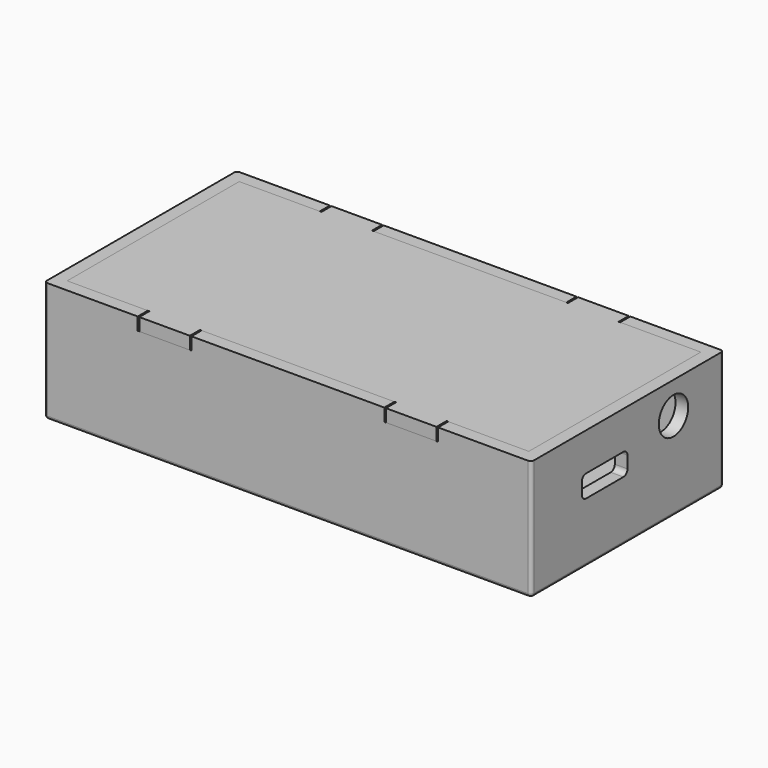
from build123d import *

# Parameters (mm, degrees)
F0_W         = 73
F0_H         = 34
F1_DEPTH     = 17
F2_T         = 2
F3_W         = 9
F3_H         = 3.5
F4_DEPTH     = 25.4
F5_R         = 2.905
F6_DEPTH     = 25.4
F7_R         = 0.8
F8_T1_DEPTH  = 37
F8_T3_DEPTH  = 19.75
F8_T5_DEPTH  = 76
F8_S9_W      = 0.51
F8_S9_H      = 0.51
F8_T10_DEPTH = 0.51
F8_S15_W     = 0.51
F8_S15_H     = 0.51
F8_T16_DEPTH = 0.51
F8_S21_W     = 0.51
F8_S21_H     = 0.51
F8_T22_DEPTH = 0.51
F8_S27_W     = 0.51
F8_S27_H     = 0.51
F8_T28_DEPTH = 0.51
F9_W         = 8.5
F9_H         = 2
F10_DEPTH    = 2
F12_DEPTH    = 2
F13_W        = 8
F13_H        = 1.5
F14_DEPTH    = 9.5
F16_DEPTH    = 1.5


# Not quite as in the source:
# - a fillet or chamfer that OpenCascade refuses, or shapes differently, is made with other operations: its cross-section is extruded or revolved along the edge and cut away or added


with BuildPart() as f1:
    # F0 (on Top) → F1 (new body)
    with BuildSketch(Plane.XY):
        with Locations((36.5, 17)):
            Rectangle(F0_W, F0_H)
    extrude(amount=F1_DEPTH)

    # F2
    f2_openings = [f1.faces().sort_by_distance(p)[0] for p in [
        (36.5, 17, 17),
    ]]
    offset(amount=F2_T, openings=f2_openings, kind=Kind.INTERSECTION)

    # F3 (on face) → F4 (cut)
    with BuildSketch(Plane.YZ.offset(75)):
        with Locations((12.5, 9.25)):
            Rectangle(F3_W, F3_H)
    extrude(amount=-F4_DEPTH, mode=Mode.SUBTRACT)

    # F5 (on face) → F6 (cut)
    with BuildSketch(Plane.YZ.offset(75)):
        with Locations((26.095, 12)):
            Circle(F5_R)
    extrude(amount=-F6_DEPTH, mode=Mode.SUBTRACT)

    # F7
    f7_edges = [f1.edges().sort_by_distance(p)[0] for p in [
        (74, 8, 7.5),
        (74, 17, 11),
        (74, 17, 7.5),
        (74, 8, 11),
    ]]
    fillet(f7_edges, radius=F7_R)

    # F8: fillet of radius 0.5 on 9 edges, made by hand

    # F8_s2 → F8_t1 (cut)
    with BuildSketch(Plane.XZ.offset(-35.5)):
        with BuildLine():
            ThreePointArc((75, -1.5), (74.8535533906, -1.8535533906), (74.5, -2))
            Line((74.5, -2), (75, -2))
            Line((75, -2), (75, -1.5))
        make_face()
        with BuildLine():
            ThreePointArc((-2, -1.5), (-1.8535533906, -1.8535533906), (-1.5, -2))
            Line((-1.5, -2), (-2, -2))
            Line((-2, -2), (-2, -1.5))
        make_face()
    extrude(amount=F8_T1_DEPTH, mode=Mode.SUBTRACT)

    # F8_s4 → F8_t3 (cut)
    with BuildSketch(Plane.XY.offset(-1.5)):
        with BuildLine():
            ThreePointArc((75, -1.5), (74.8535533906, -1.8535533906), (74.5, -2))
            Line((74.5, -2), (75, -2))
            Line((75, -2), (75, -1.5))
        make_face()
        with BuildLine():
            ThreePointArc((75, 35.5), (74.8535533906, 35.8535533906), (74.5, 36))
            Line((74.5, 36), (75, 36))
            Line((75, 36), (75, 35.5))
        make_face()
        with BuildLine():
            ThreePointArc((-1.5, 36), (-1.8535533906, 35.8535533906), (-2, 35.5))
            Line((-2, 35.5), (-2, 36))
            Line((-2, 36), (-1.5, 36))
        make_face()
        with BuildLine():
            ThreePointArc((-2, -1.5), (-1.8535533906, -1.8535533906), (-1.5, -2))
            Line((-1.5, -2), (-2, -2))
            Line((-2, -2), (-2, -1.5))
        make_face()
    extrude(amount=F8_T3_DEPTH, mode=Mode.SUBTRACT)

    # F8_s6 → F8_t5 (cut)
    with BuildSketch(Plane.YZ.offset(-1.5)):
        with BuildLine():
            ThreePointArc((36, -1.5), (35.8535533906, -1.8535533906), (35.5, -2))
            Line((35.5, -2), (36, -2))
            Line((36, -2), (36, -1.5))
        make_face()
        with BuildLine():
            ThreePointArc((-2, -1.5), (-1.8535533906, -1.8535533906), (-1.5, -2))
            Line((-1.5, -2), (-2, -2))
            Line((-2, -2), (-2, -1.5))
        make_face()
    extrude(amount=F8_T5_DEPTH, mode=Mode.SUBTRACT)


with BuildPart() as f8_tool8:
    # F8_s9 → F8_t10 (new body)
    with BuildSketch(Plane.XZ.offset(1.5)):
        with Locations((74.755, -1.755)):
            Rectangle(F8_S9_W, F8_S9_H)
    extrude(amount=F8_T10_DEPTH)

    # F8_s11 → F8_t12 (revolve, cut)
    with BuildSketch(Plane(origin=(74.5, -1.5, -1.5), x_dir=(-0.7071067812, 0, 0.7071067812), z_dir=(0.7071067812, 0, 0.7071067812))):
        with BuildLine():
            ThreePointArc((0, -0.5), (0.5, 0), (0, 0.5))
            Line((0, 0.5), (0, -0.5))
        make_face()
    revolve(axis=Axis((74.5, -1.5, -1.5), (0, -1, 0)), mode=Mode.SUBTRACT)


with BuildPart() as f1_1:
    add(f1.part)

    # F8_t7: cut F8_tool8
    add(f8_tool8.part, mode=Mode.SUBTRACT)


with BuildPart() as f8_tool14:
    # F8_s15 → F8_t16 (new body)
    with BuildSketch(Plane.XZ.offset(-35.5)):
        with Locations((74.755, -1.755)):
            Rectangle(F8_S15_W, F8_S15_H)
    extrude(amount=-F8_T16_DEPTH)

    # F8_s17 → F8_t18 (revolve, cut)
    with BuildSketch(Plane(origin=(74.5, 35.5, -1.5), x_dir=(-0.7071067812, 0, 0.7071067812), z_dir=(-0.7071067812, 0, -0.7071067812))):
        with BuildLine():
            ThreePointArc((0, -0.5), (0.5, 0), (0, 0.5))
            Line((0, 0.5), (0, -0.5))
        make_face()
    revolve(axis=Axis((74.5, 35.5, -1.5), (0, 1, 0)), mode=Mode.SUBTRACT)


with BuildPart() as f1_2:
    add(f1_1.part)

    # F8_t13: cut F8_tool14
    add(f8_tool14.part, mode=Mode.SUBTRACT)


with BuildPart() as f8_tool20:
    # F8_s21 → F8_t22 (new body)
    with BuildSketch(Plane.XZ.offset(-35.5)):
        with Locations((-1.755, -1.755)):
            Rectangle(F8_S21_W, F8_S21_H)
    extrude(amount=-F8_T22_DEPTH)

    # F8_s23 → F8_t24 (revolve, cut)
    with BuildSketch(Plane(origin=(-1.5, 35.5, -1.5), x_dir=(0.7071067812, 0, 0.7071067812), z_dir=(-0.7071067812, 0, 0.7071067812))):
        with BuildLine():
            ThreePointArc((0, -0.5), (0.5, 0), (0, 0.5))
            Line((0, 0.5), (0, -0.5))
        make_face()
    revolve(axis=Axis((-1.5, 35.5, -1.5), (0, 1, 0)), mode=Mode.SUBTRACT)


with BuildPart() as f1_3:
    add(f1_2.part)

    # F8_t19: cut F8_tool20
    add(f8_tool20.part, mode=Mode.SUBTRACT)


with BuildPart() as f8_tool26:
    # F8_s27 → F8_t28 (new body)
    with BuildSketch(Plane.YZ.offset(-1.5)):
        with Locations((-1.755, -1.755)):
            Rectangle(F8_S27_W, F8_S27_H)
    extrude(amount=-F8_T28_DEPTH)

    # F8_s29 → F8_t30 (revolve, cut)
    with BuildSketch(Plane(origin=(-1.5, -1.5, -1.5), x_dir=(0, 0.7071067812, 0.7071067812), z_dir=(0, -0.7071067812, 0.7071067812))):
        with BuildLine():
            ThreePointArc((0, -0.5), (0.5, 0), (0, 0.5))
            Line((0, 0.5), (0, -0.5))
        make_face()
    revolve(axis=Axis((-1.5, -1.5, -1.5), (-1, 0, 0)), mode=Mode.SUBTRACT)


with BuildPart() as f1_4:
    add(f1_3.part)

    # F8_t25: cut F8_tool26
    add(f8_tool26.part, mode=Mode.SUBTRACT)

    # F9 (on face) → F10 (cut)
    with BuildSketch(Plane.XY.offset(17)):
        with Locations((17, 35)):
            Rectangle(F9_W, F9_H)
        with Locations((56, 35)):
            Rectangle(F9_W, F9_H)
        with Locations((56, -1)):
            Rectangle(F9_W, F9_H)
        with Locations((17, -1)):
            Rectangle(F9_W, F9_H)
    extrude(amount=-F10_DEPTH, mode=Mode.SUBTRACT)

    # F13 (on face) → F14 (join)
    with BuildSketch(Plane.XY):
        with Locations((4, 7.25)):
            Rectangle(F13_W, F13_H)
    extrude(amount=F14_DEPTH)

    # F15 (on face) → F16 (join)
    with BuildSketch(Plane.XZ.offset(-6.5)):
        Polygon((0, 12.5), (0, 9.5), (9, 9.5), (8, 12.5), align=None)
    extrude(amount=-F16_DEPTH)


with BuildPart() as f12:
    # F11 (on face) → F12 (new body)
    with BuildSketch(Plane.XY.offset(17)):
        Polygon((0, 34), (0, 0), (13, 0), (13, -2), (21, -2), (21, 0), (52, 0), (52, -2), (60, -2), (60, 0), (73, 0), (73, 34), (60, 34), (60, 36), (52, 36), (52, 34), (21, 34), (21, 36), (13, 36), (13, 34), align=None)
    extrude(amount=-F12_DEPTH)


solid = Compound([f1_4.part, f12.part])
